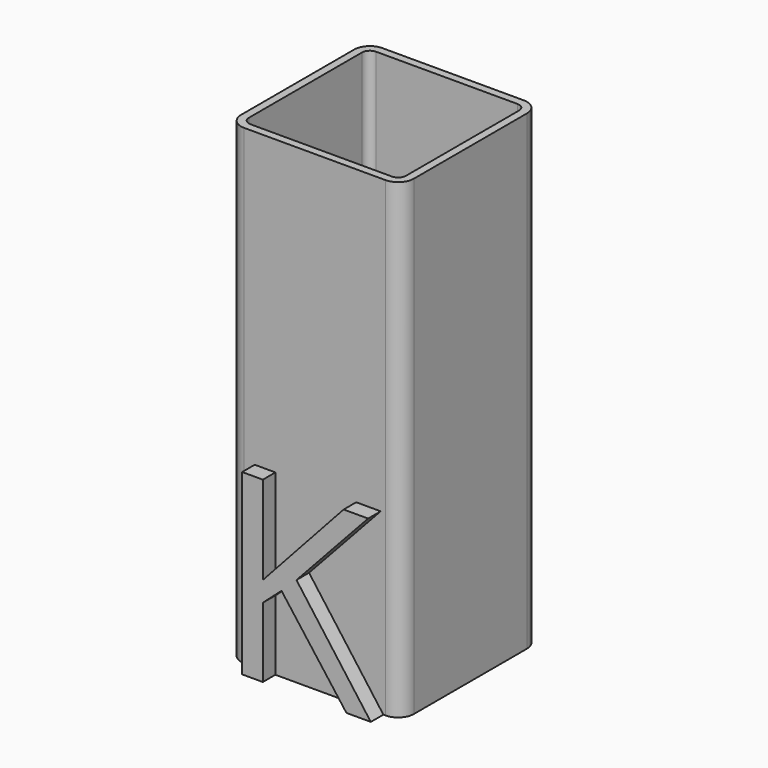
from build123d import *

# Parameters (mm, degrees)
F1_DEPTH     = 150
F2_T         = -2.5
F3_TEXT_SIZE = 79.429847381
F4_DEPTH     = 5


# Not quite as in the source:
# - Text() gives the source's letters only with a copy of the font that has no kerning and outlines rounded to 1/6400 em; it was checked with that copy


with BuildPart() as f1:
    # F0 (on Top) → F1 (new body)
    with BuildSketch(Plane.XY):
        with BuildLine():
            Line((-22.5, -27.5), (22.5, -27.5))
            ThreePointArc((22.5, -27.5), (26.0355339059, -26.0355339059), (27.5, -22.5))
            Line((27.5, -22.5), (27.5, 22.5))
            ThreePointArc((27.5, 22.5), (26.0355339059, 26.0355339059), (22.5, 27.5))
            Line((22.5, 27.5), (-22.5, 27.5))
            ThreePointArc((-22.5, 27.5), (-26.0355339059, 26.0355339059), (-27.5, 22.5))
            Line((-27.5, 22.5), (-27.5, -22.5))
            ThreePointArc((-27.5, -22.5), (-26.0355339059, -26.0355339059), (-22.5, -27.5))
        make_face()
    extrude(amount=F1_DEPTH)

    # F2
    f2_openings = [f1.faces().sort_by_distance(p)[0] for p in [
        (0, 0, 150),
    ]]
    offset(amount=F2_T, openings=f2_openings)

    # F3 (on face) → F4 (join)
    with BuildSketch(Plane.XZ.offset(27.5)):
        with Locations((-26.9502989981, 0)):
            Text('K', F3_TEXT_SIZE, font='Open Sans', text_align=(TextAlign.LEFT, TextAlign.BOTTOM))
    extrude(amount=F4_DEPTH)


solid = f1.part
